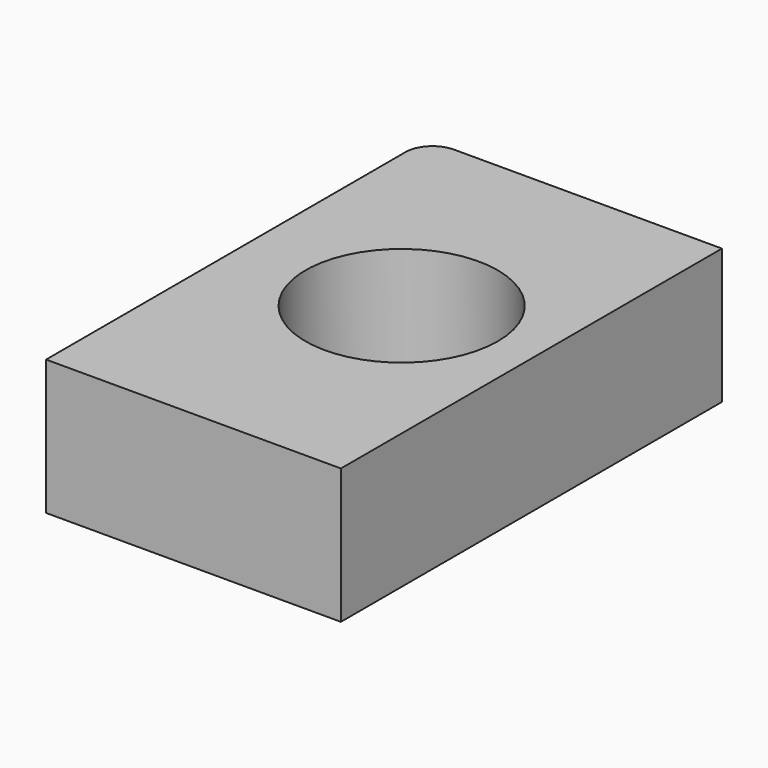
from build123d import *

# Parameters (mm, degrees)
F0_W     = 55.4524268955
F0_H     = 89.5769931376
F1_DEPTH = 25.4
F2_R     = 5.08
F3_R     = 18.0864233447
F4_DEPTH = 25.4
F5_T     = -2.54


with BuildPart() as f1:
    # F0 (on Top) → F1 (new body)
    with BuildSketch(Plane.XY):
        with Locations((-2.3697623983, -1.1848751456)):
            Rectangle(F0_W, F0_H)
    extrude(amount=-F1_DEPTH)

    # F2
    f2_edges = [f1.edges().sort_by_distance(p)[0] for p in [
        (-30.095976, 43.603621, -12.7),
    ]]
    fillet(f2_edges, radius=F2_R)

    # F3 (on face) → F4 (cut)
    with BuildSketch(Plane(origin=(0, 0, -25.4), x_dir=(1, 0, 0), z_dir=(0, 0, -1))):
        Circle(F3_R)
    extrude(amount=-F4_DEPTH, mode=Mode.SUBTRACT)

    # F5
    f5_openings = [f1.faces().sort_by_distance(p)[0] for p in [
        (0.170238, 42.550103, -25.4),
    ]]
    offset(amount=F5_T, openings=f5_openings)


solid = f1.part
